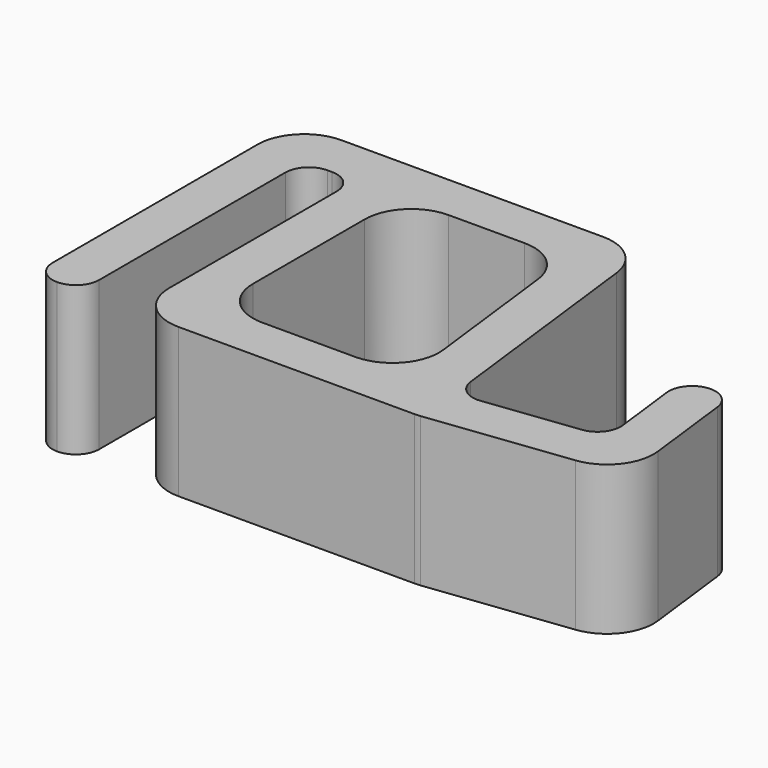
from build123d import *

# Parameters (mm, degrees)
F0_W     = 5
F0_H     = 30
F1_DEPTH = 16
F2_R     = 5
F3_R     = 2.49999


# Not quite as in the source:
# - a fillet or chamfer is up to 0.001 mm smaller than in the source, because OpenCascade refuses the exact size
# - a feature names something its author has since deleted; it is built from what else it names


with BuildPart() as f1:
    # F0 (on Top) → F1 (new body)
    with BuildSketch(Plane.XY):
        with Locations((-13, -119.1857503612)):
            Rectangle(F0_W, F0_H)
        Polygon((-15.5, -99.1857503612), (-15.5, -104.1857503612), (-10.5, -104.1857503612), (-5, -104.1857503612), (0, -104.1857503612), (0, -99.1857503612), align=None)
        Polygon((0, -104.1857503612), (-5, -104.1857503612), (-5, -134.1857503612), (0, -134.1857503612), (0, -129.1857503612), align=None)
        Polygon((22.0267780379, -99.1857503612), (0, -99.1857503612), (0, -104.1857503612), (17.5957249839, -104.1857503612), (20.6230915981, -129.1857503612), (0, -129.1857503612), (0, -134.1857503612), (25.6551948256, -134.1857503612), (46.11123117, -131.7086335017), (44.067551515, -114.8319225227), (39.1038129917, -115.4330047742), (40.5464103953, -127.3459772299), (25.6551948256, -129.1492239844), align=None)
    extrude(amount=F1_DEPTH)

    # F2
    f2_edges = [f1.edges().sort_by_distance(p)[0] for p in [
        (-15.5, -99.18575, 8),
        (0, -104.18575, 8),
        (17.595725, -104.18575, 8),
        (20.623092, -129.18575, 8),
        (0, -129.18575, 8),
        (-5, -134.18575, 8),
        (22.026778, -99.18575, 8),
        (25.655195, -134.18575, 8),
        (46.111231, -131.708634, 8),
    ]]
    fillet(f2_edges, radius=F2_R)

    # F3 (radius 2.5 in the source; OpenCascade refuses exactly that, so slightly less here)
    f3_edges = [f1.edges().sort_by_distance(p)[0] for p in [
        (44.067552, -114.831923, 8),
        (39.103813, -115.433005, 8),
        (-15.5, -134.18575, 8),
        (-10.5, -134.18575, 8),
        (-10.5, -104.18575, 8),
        (-5, -104.18575, 8),
        (25.655195, -129.149224, 8),
        (40.54641, -127.345977, 8),
    ]]
    fillet(f3_edges, radius=F3_R)


solid = f1.part
